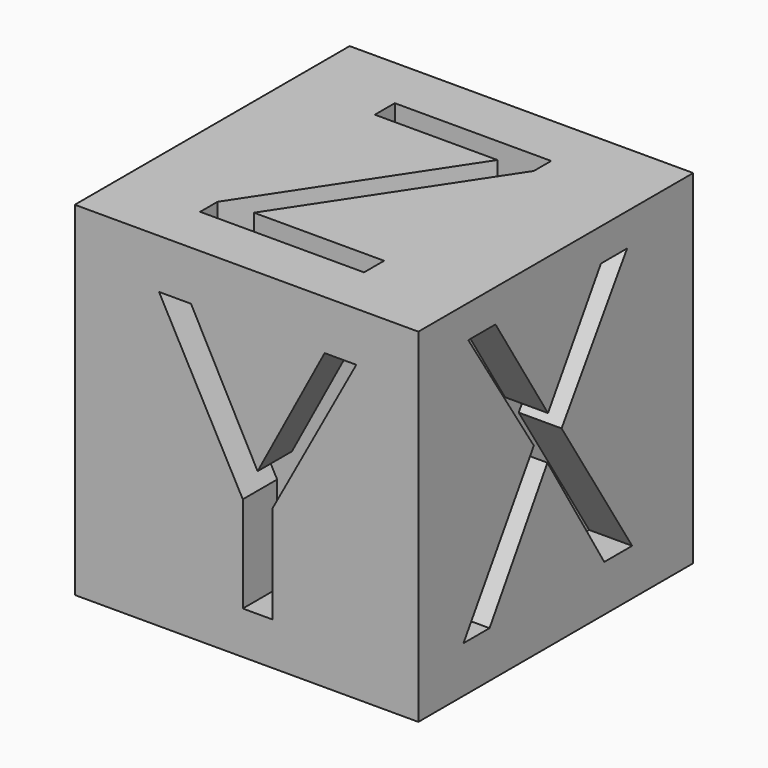
from build123d import *

# Parameters (mm, degrees)
F0_W         = 25.4
F0_H         = 25.4
F1_DEPTH     = 25.4
F2_TEXT_SIZE = 24.6886590806
F3_DEPTH     = 3.175
F4_TEXT_SIZE = 26.0420169474
F5_DEPTH     = 3.175
F6_TEXT_SIZE = 27.3797916533
F7_DEPTH     = 3.175


# Not quite as in the source:
# - Text() gives the source's letters only with a copy of the font that has no kerning and outlines rounded to 1/6400 em; it was checked with that copy


with BuildPart() as f1:
    # F0 (on Top) → F1 (new body)
    with BuildSketch(Plane.XY):
        Rectangle(F0_W, F0_H)
    extrude(amount=F1_DEPTH)

    # F2 (on face) → F3 (cut)
    with BuildSketch(Plane.XY.offset(25.4)):
        with Locations((-7.4836327694, -8.8712070137)):
            Text('Z', F2_TEXT_SIZE, font='Open Sans', text_align=(TextAlign.LEFT, TextAlign.BOTTOM))
    extrude(amount=-F3_DEPTH, mode=Mode.SUBTRACT)

    # F4 (on face) → F5 (cut)
    with BuildSketch(Plane.XZ.offset(12.7)):
        with Locations((-6.4725680277, 3.1592454761)):
            Text('Y', F4_TEXT_SIZE, font='Open Sans', text_align=(TextAlign.LEFT, TextAlign.BOTTOM))
    extrude(amount=-F5_DEPTH, mode=Mode.SUBTRACT)

    # F6 (on face) → F7 (cut)
    with BuildSketch(Plane.YZ.offset(12.7)):
        with Locations((-8.6358897388, 3.4276770893)):
            Text('X', F6_TEXT_SIZE, font='Open Sans', text_align=(TextAlign.LEFT, TextAlign.BOTTOM))
    extrude(amount=-F7_DEPTH, mode=Mode.SUBTRACT)


solid = f1.part
